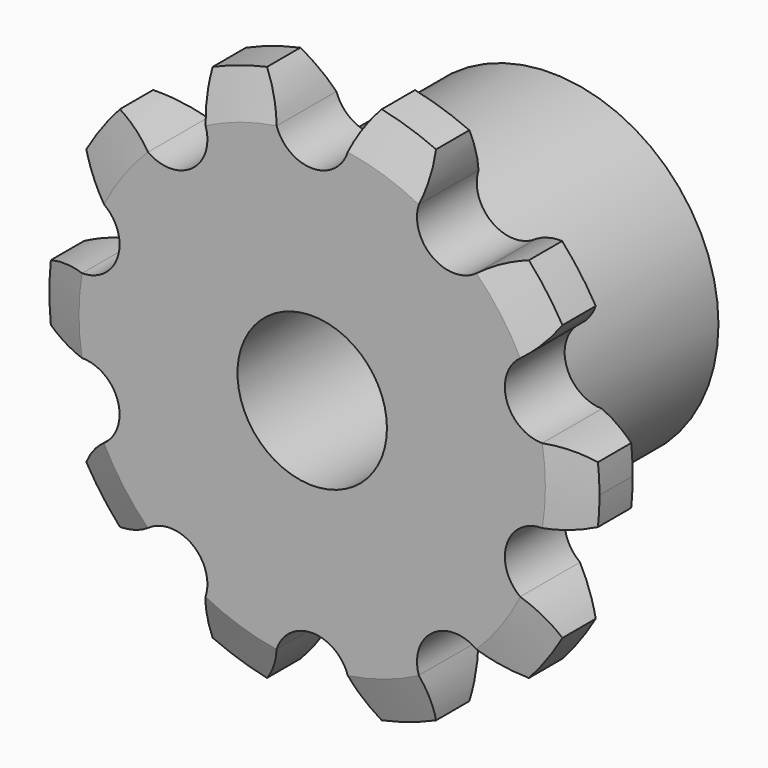
from build123d import *

# Parameters (mm, degrees)
F0_R         = 7.0995158286
F0_R_2       = 3.175
F1_DEPTH     = 3.175
F2_DEPTH     = 9.525
F3_T2_ANGLE  = 57.1640564586
F3_T4_ANGLE  = 57.1640564586
F3_T6_ANGLE  = 57.1640564586
F3_T8_ANGLE  = 57.1640564586
F3_T10_ANGLE = 57.1640564586
F3_T12_ANGLE = 57.1640564586
F3_T14_ANGLE = 57.1640564586
F3_T16_ANGLE = 57.1640564586
F3_T18_ANGLE = 57.1640564586
F3_T20_ANGLE = 57.1640564586
F4_C1_SIZE2  = 0.762
F4_C1_SIZE   = 1.7951595028
F4_C2_SIZE2  = 0.762
F4_C2_SIZE   = 1.7951595028
F4_C3_SIZE2  = 0.762
F4_C3_SIZE   = 1.7951595028
F4_C4_SIZE2  = 0.762
F4_C4_SIZE   = 1.7951595028
F4_C5_SIZE2  = 0.762
F4_C5_SIZE   = 1.7951595028
F4_C6_SIZE2  = 0.762
F4_C6_SIZE   = 1.7951595028
F4_C7_SIZE2  = 0.762
F4_C7_SIZE   = 1.7951595028
F4_C8_SIZE2  = 0.762
F4_C8_SIZE   = 1.7951595028
F4_C9_SIZE2  = 0.762
F4_C9_SIZE   = 1.7951595028
F4_C10_SIZE2 = 0.762
F4_C10_SIZE  = 1.7951595028


# Not quite as in the source:
# - a fillet or chamfer that OpenCascade refuses, or shapes differently, is made with other operations: its cross-section is extruded or revolved along the edge and cut away or added


with BuildPart() as f1:
    # F0 (on Front) → F1 (new body)
    with BuildSketch(Plane.XZ):
        with BuildLine():
            ThreePointArc((6.9723179665, 7.0279434357), (5.1060997905, 7.0279434357), (4.5294066589, 8.8028223929))
            ThreePointArc((4.5294066589, 8.8028223929), (4.7311609803, 9.7290600297), (4.7454701141, 10.6769082321))
            ThreePointArc((4.7454701141, 10.6769082321), (3.6105545623, 11.1121443364), (2.4365632303, 11.4271175554))
            ThreePointArc((2.4365632303, 11.4271175554), (1.8910083679, 10.6518815537), (1.5098022196, 9.78395135))
            ThreePointArc((1.5098022196, 9.78395135), (0, 8.6870158286), (-1.5098022196, 9.78395135))
            ThreePointArc((-1.5098022196, 9.78395135), (-1.8910083679, 10.6518815537), (-2.4365632303, 11.4271175554))
            ThreePointArc((-2.4365632303, 11.4271175554), (-3.6105545623, 11.1121443364), (-4.7454701141, 10.6769082321))
            ThreePointArc((-4.7454701141, 10.6769082321), (-4.7311609803, 9.7290600297), (-4.5294066589, 8.8028223929))
            ThreePointArc((-4.5294066589, 8.8028223929), (-4.4712536378, 8.5605976275), (-4.4517088785, 8.3122579143))
            ThreePointArc((-4.4517088785, 8.3122579143), (-5.3184989601, 6.8977850571), (-6.9723179665, 7.0279434357))
            ThreePointArc((-6.9723179665, 7.0279434357), (-7.7908767926, 7.5060463684), (-8.6879122365, 7.812556366))
            ThreePointArc((-8.6879122365, 7.812556366), (-9.4525545623, 6.8676828878), (-10.1148951675, 5.8484828589))
            ThreePointArc((-10.1148951675, 5.8484828589), (-9.5461876403, 5.0900682529), (-8.8385361425, 4.4593144786))
            ThreePointArc((-8.8385361425, 4.4593144786), (-8.3571723734, 3.8957099183), (-8.1841452305, 3.175))
            ThreePointArc((-8.1841452305, 3.175), (-8.6491132154, 2.0524679849), (-9.7716452305, 1.5875))
            ThreePointArc((-9.7716452305, 1.5875), (-10.7148950847, 1.4931565915), (-11.6207740596, 1.2138641838))
            ThreePointArc((-11.6207740596, 1.2138641838), (-11.684, 0), (-11.6207740596, -1.2138641838))
            ThreePointArc((-11.6207740596, -1.2138641838), (-10.7148950847, -1.4931565915), (-9.7716452305, -1.5875))
            ThreePointArc((-9.7716452305, -1.5875), (-8.6491132154, -2.0524679849), (-8.1841452305, -3.175))
            ThreePointArc((-8.1841452305, -3.175), (-8.3571723734, -3.8957099183), (-8.8385361425, -4.4593144786))
            ThreePointArc((-8.8385361425, -4.4593144786), (-9.5461876403, -5.0900682529), (-10.1148951675, -5.8484828589))
            ThreePointArc((-10.1148951675, -5.8484828589), (-9.4525545623, -6.8676828878), (-8.6879122365, -7.812556366))
            ThreePointArc((-8.6879122365, -7.812556366), (-7.7908767926, -7.5060463684), (-6.9723179665, -7.0279434357))
            ThreePointArc((-6.9723179665, -7.0279434357), (-5.3184989601, -6.8977850571), (-4.4517088785, -8.3122579143))
            ThreePointArc((-4.4517088785, -8.3122579143), (-4.4712536378, -8.5605976275), (-4.5294066589, -8.8028223929))
            ThreePointArc((-4.5294066589, -8.8028223929), (-4.7311609803, -9.7290600297), (-4.7454701141, -10.6769082321))
            ThreePointArc((-4.7454701141, -10.6769082321), (-3.6105545623, -11.1121443364), (-2.4365632303, -11.4271175554))
            ThreePointArc((-2.4365632303, -11.4271175554), (-1.8910083679, -10.6518815537), (-1.5098022196, -9.78395135))
            ThreePointArc((-1.5098022196, -9.78395135), (0, -8.6870158286), (1.5098022196, -9.78395135))
            ThreePointArc((1.5098022196, -9.78395135), (1.8910083679, -10.6518815537), (2.4365632303, -11.4271175554))
            ThreePointArc((2.4365632303, -11.4271175554), (3.6105545623, -11.1121443364), (4.7454701141, -10.6769082321))
            ThreePointArc((4.7454701141, -10.6769082321), (4.7311609803, -9.7290600297), (4.5294066589, -8.8028223929))
            ThreePointArc((4.5294066589, -8.8028223929), (5.1060997905, -7.0279434357), (6.9723179665, -7.0279434357))
            ThreePointArc((6.9723179665, -7.0279434357), (7.7908767926, -7.5060463684), (8.6879122365, -7.812556366))
            ThreePointArc((8.6879122365, -7.812556366), (9.4525545623, -6.8676828878), (10.1148951675, -5.8484828589))
            ThreePointArc((10.1148951675, -5.8484828589), (9.5461876403, -5.0900682529), (8.8385361425, -4.4593144786))
            ThreePointArc((8.8385361425, -4.4593144786), (8.2618430109, -2.6844355214), (9.7716452305, -1.5875))
            ThreePointArc((9.7716452305, -1.5875), (10.7148950847, -1.4931565915), (11.6207740596, -1.2138641838))
            ThreePointArc((11.6207740596, -1.2138641838), (11.6681828086, -0.6077548388), (11.684, 0))
            ThreePointArc((11.684, 0), (11.6681828086, 0.6077548388), (11.6207740596, 1.2138641838))
            ThreePointArc((11.6207740596, 1.2138641838), (10.7148950847, 1.4931565915), (9.7716452305, 1.5875))
            ThreePointArc((9.7716452305, 1.5875), (8.2618430109, 2.6844355214), (8.8385361425, 4.4593144786))
            ThreePointArc((8.8385361425, 4.4593144786), (9.5461876403, 5.0900682529), (10.1148951675, 5.8484828589))
            ThreePointArc((10.1148951675, 5.8484828589), (9.4525545623, 6.8676828878), (8.6879122365, 7.812556366))
            ThreePointArc((8.6879122365, 7.812556366), (7.7908767926, 7.5060463684), (6.9723179665, 7.0279434357))
        make_face()
        Circle(F0_R, mode=Mode.SUBTRACT)
        Circle(F0_R)
        Circle(F0_R_2, mode=Mode.SUBTRACT)
    extrude(amount=F1_DEPTH)

    # F0 (on Front) → F2 (join)
    with BuildSketch(Plane.XZ):
        Circle(F0_R)
        Circle(F0_R_2, mode=Mode.SUBTRACT)
    extrude(amount=-F2_DEPTH)

    # F3: chamfer of 1.778 x 0.6471390765 on 10 edges, made by hand

    # F3_s1 → F3_t2 (revolve, cut)
    with BuildSketch(Plane(origin=(0, 0, 0), x_dir=(0, 1, 0), z_dir=(0.9829930002, 0, -0.1836430276))):
        Polygon((-2.5278609235, 11.684), (-3.175, 9.906), (-3.175, 11.684), align=None)
    revolve(axis=Axis((0, -3.175, 0), (0, -1, 0)), revolution_arc=F3_T2_ANGLE, mode=Mode.SUBTRACT)

    # F3_s3 → F3_t4 (revolve, cut)
    with BuildSketch(Plane(origin=(0, 0, 0), x_dir=(0, 1, 0), z_dir=(0.6873153792, 0, -0.7263591188))):
        Polygon((-2.5278609235, 11.684), (-3.175, 9.906), (-3.175, 11.684), align=None)
    revolve(axis=Axis((0, -3.175, 0), (0, -1, 0)), revolution_arc=F3_T4_ANGLE, mode=Mode.SUBTRACT)

    # F3_s5 → F3_t6 (revolve, cut)
    with BuildSketch(Plane(origin=(0, 0, 0), x_dir=(0, 1, 0), z_dir=(0.1291066443, 0, -0.9916307147))):
        Polygon((-2.5278609235, 11.684), (-3.175, 9.906), (-3.175, 11.684), align=None)
    revolve(axis=Axis((0, -3.175, 0), (0, -1, 0)), revolution_arc=F3_T6_ANGLE, mode=Mode.SUBTRACT)

    # F3_s7 → F3_t8 (revolve, cut)
    with BuildSketch(Plane(origin=(0, 0, 0), x_dir=(0, 1, 0), z_dir=(-0.4784164405, 0, -0.8781330819))):
        Polygon((-2.5278609235, 11.684), (-3.175, 9.906), (-3.175, 11.684), align=None)
    revolve(axis=Axis((0, -3.175, 0), (0, -1, 0)), revolution_arc=F3_T8_ANGLE, mode=Mode.SUBTRACT)

    # F3_s9 → F3_t10 (revolve, cut)
    with BuildSketch(Plane(origin=(0, 0, 0), x_dir=(0, 1, 0), z_dir=(-0.9032007058, 0, -0.4292184584))):
        Polygon((-2.5278609235, 11.684), (-3.175, 9.906), (-3.175, 11.684), align=None)
    revolve(axis=Axis((0, -3.175, 0), (0, -1, 0)), revolution_arc=F3_T10_ANGLE, mode=Mode.SUBTRACT)

    # F3_s11 → F3_t12 (revolve, cut)
    with BuildSketch(Plane(origin=(0, 0, 0), x_dir=(0, 1, 0), z_dir=(-0.9829930002, 0, 0.1836430276))):
        Polygon((-2.5278609235, 11.684), (-3.175, 9.906), (-3.175, 11.684), align=None)
    revolve(axis=Axis((0, -3.175, 0), (0, -1, 0)), revolution_arc=F3_T12_ANGLE, mode=Mode.SUBTRACT)

    # F3_s13 → F3_t14 (revolve, cut)
    with BuildSketch(Plane(origin=(0, 0, 0), x_dir=(0, 1, 0), z_dir=(-0.6873153792, 0, 0.7263591188))):
        Polygon((-2.5278609235, 11.684), (-3.175, 9.906), (-3.175, 11.684), align=None)
    revolve(axis=Axis((0, -3.175, 0), (0, -1, 0)), revolution_arc=F3_T14_ANGLE, mode=Mode.SUBTRACT)

    # F3_s15 → F3_t16 (revolve, cut)
    with BuildSketch(Plane(origin=(0, 0, 0), x_dir=(0, 1, 0), z_dir=(-0.1291066443, 0, 0.9916307147))):
        Polygon((-2.5278609235, 11.684), (-3.175, 9.906), (-3.175, 11.684), align=None)
    revolve(axis=Axis((0, -3.175, 0), (0, -1, 0)), revolution_arc=F3_T16_ANGLE, mode=Mode.SUBTRACT)

    # F3_s17 → F3_t18 (revolve, cut)
    with BuildSketch(Plane(origin=(0, 0, 0), x_dir=(0, 1, 0), z_dir=(0.4784164405, 0, 0.8781330819))):
        Polygon((-2.5278609235, 11.684), (-3.175, 9.906), (-3.175, 11.684), align=None)
    revolve(axis=Axis((0, -3.175, 0), (0, -1, 0)), revolution_arc=F3_T18_ANGLE, mode=Mode.SUBTRACT)

    # F3_s19 → F3_t20 (revolve, cut)
    with BuildSketch(Plane(origin=(0, 0, 0), x_dir=(0, 1, 0), z_dir=(0.9032007058, 0, 0.4292184584))):
        Polygon((-2.5278609235, 11.684), (-3.175, 9.906), (-3.175, 11.684), align=None)
    revolve(axis=Axis((0, -3.175, 0), (0, -1, 0)), revolution_arc=F3_T20_ANGLE, mode=Mode.SUBTRACT)

    # F4: chamfer of 0.762 x 1.7951595028 on 10 edges, made by hand

    # F4_c1
    f4_c1_edges = [f1.edges().sort_by_distance(p)[0] for p in [
        (-11.684, 0, 0),
    ]]
    f4_c1_side = f1.faces().sort_by_distance((-11.66876, 0, 0))[0]
    chamfer(f4_c1_edges, length=F4_C1_SIZE, length2=F4_C1_SIZE2, reference=f4_c1_side)

    # F4_c2
    f4_c2_edges = [f1.edges().sort_by_distance(p)[0] for p in [
        (-9.4525545623, 0, 6.8676828878),
    ]]
    f4_c2_side = f1.faces().sort_by_distance((-9.4402251433, 0, 6.8587250405))[0]
    chamfer(f4_c2_edges, length=F4_C2_SIZE, length2=F4_C2_SIZE2, reference=f4_c2_side)

    # F4_c3
    f4_c3_edges = [f1.edges().sort_by_distance(p)[0] for p in [
        (9.4525545623, 0, 6.8676828878),
    ]]
    f4_c3_side = f1.faces().sort_by_distance((9.4402251433, 0, 6.8587250405))[0]
    chamfer(f4_c3_edges, length=F4_C3_SIZE, length2=F4_C3_SIZE2, reference=f4_c3_side)

    # F4_c4
    f4_c4_edges = [f1.edges().sort_by_distance(p)[0] for p in [
        (-9.4525545623, 0, -6.8676828878),
    ]]
    f4_c4_side = f1.faces().sort_by_distance((-9.4402251433, 0, -6.8587250405))[0]
    chamfer(f4_c4_edges, length=F4_C4_SIZE, length2=F4_C4_SIZE2, reference=f4_c4_side)

    # F4_c5
    f4_c5_edges = [f1.edges().sort_by_distance(p)[0] for p in [
        (9.4525545623, 0, -6.8676828878),
    ]]
    f4_c5_side = f1.faces().sort_by_distance((9.4402251433, 0, -6.8587250405))[0]
    chamfer(f4_c5_edges, length=F4_C5_SIZE, length2=F4_C5_SIZE2, reference=f4_c5_side)

    # F4_c6
    f4_c6_edges = [f1.edges().sort_by_distance(p)[0] for p in [
        (11.684, 0, 0),
    ]]
    f4_c6_side = f1.faces().sort_by_distance((11.66876, 0, 0))[0]
    chamfer(f4_c6_edges, length=F4_C6_SIZE, length2=F4_C6_SIZE2, reference=f4_c6_side)

    # F4_c7
    f4_c7_edges = [f1.edges().sort_by_distance(p)[0] for p in [
        (3.6105545623, 0, -11.1121443364),
    ]]
    f4_c7_side = f1.faces().sort_by_distance((3.6058451433, 0, -11.0976502351))[0]
    chamfer(f4_c7_edges, length=F4_C7_SIZE, length2=F4_C7_SIZE2, reference=f4_c7_side)

    # F4_c8
    f4_c8_edges = [f1.edges().sort_by_distance(p)[0] for p in [
        (-3.6105545623, 0, -11.1121443364),
    ]]
    f4_c8_side = f1.faces().sort_by_distance((-3.6058451433, 0, -11.0976502351))[0]
    chamfer(f4_c8_edges, length=F4_C8_SIZE, length2=F4_C8_SIZE2, reference=f4_c8_side)

    # F4_c9
    f4_c9_edges = [f1.edges().sort_by_distance(p)[0] for p in [
        (3.6105545623, 0, 11.1121443364),
    ]]
    f4_c9_side = f1.faces().sort_by_distance((3.6058451433, 0, 11.0976502351))[0]
    chamfer(f4_c9_edges, length=F4_C9_SIZE, length2=F4_C9_SIZE2, reference=f4_c9_side)

    # F4_c10
    f4_c10_edges = [f1.edges().sort_by_distance(p)[0] for p in [
        (-3.6105545623, 0, 11.1121443364),
    ]]
    f4_c10_side = f1.faces().sort_by_distance((-3.6058451433, 0, 11.0976502351))[0]
    chamfer(f4_c10_edges, length=F4_C10_SIZE, length2=F4_C10_SIZE2, reference=f4_c10_side)


solid = f1.part
